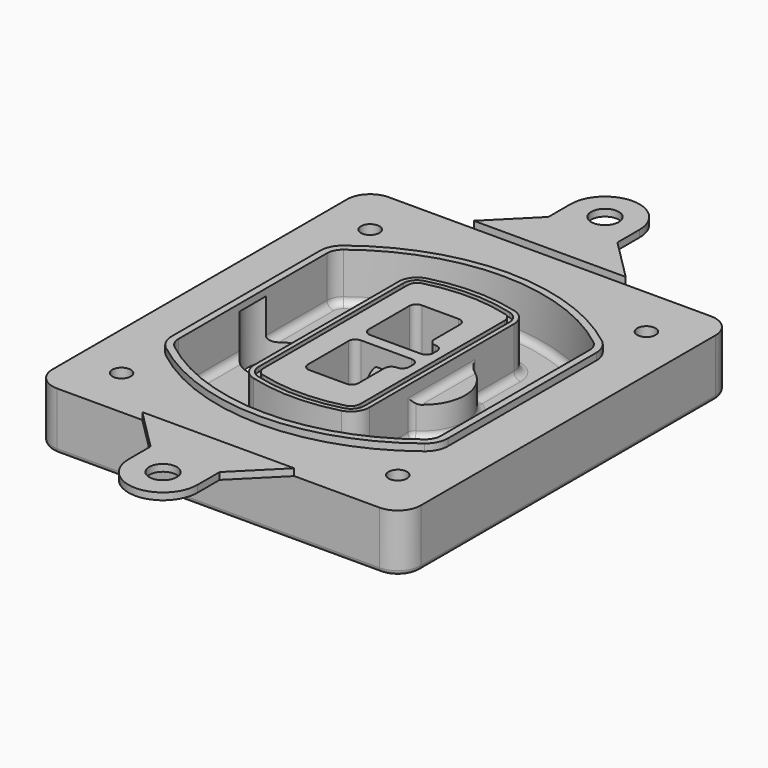
from build123d import *

# Parameters (mm, degrees)
F0_R      = 4
F1_DEPTH  = 25
F2_DEPTH  = 3
F3_DEPTH  = 18
F5_DEPTH  = 21
F6_DEPTH  = 2
F8_DEPTH  = 20
F9_DEPTH  = 16
F10_DEPTH = 25
F7_R      = 6
F7_R_2    = 4
F11_DEPTH = 6
F13_DEPTH = 9
F14_R     = 3
F15_R     = 2
F16_R     = 6
F17_DEPTH = 3
F18_DEPTH = 3


# Not quite as in the source:
# - a feature names something its author has since deleted; it is built from what else it names


with BuildPart() as f1:
    # F0 (on Top) → F1 (new body)
    with BuildSketch(Plane.XY):
        with BuildLine():
            ThreePointArc((-80, -80), (-77.0710678119, -87.0710678119), (-70, -90))
            Line((-70, -90), (70, -90))
            ThreePointArc((70, -90), (77.0710678119, -87.0710678119), (80, -80))
            Line((80, -80), (80, 80))
            ThreePointArc((80, 80), (77.0710678119, 87.0710678119), (70, 90))
            Line((70, 90), (-70, 90))
            ThreePointArc((-70, 90), (-77.0710678119, 87.0710678119), (-80, 80))
            Line((-80, 80), (-80, -80))
        make_face()
        with Locations((-60, -67.5)):
            Circle(F0_R, mode=Mode.SUBTRACT)
        with Locations((60, -67.5)):
            Circle(F0_R, mode=Mode.SUBTRACT)
        with Locations((-60, 67.5)):
            Circle(F0_R, mode=Mode.SUBTRACT)
        with BuildLine():
            ThreePointArc((-64, 40.2934422872), (-62.5820384798, 46.4328484224), (-58.6153846154, 51.3286200352))
            ThreePointArc((-58.6153846154, 51.3286200352), (0, 71.5), (58.6153846154, 51.3286200352))
            ThreePointArc((58.6153846154, 51.3286200352), (62.5820384798, 46.4328484224), (64, 40.2934422872))
            Line((64, 40.2934422872), (64, -40.2934422872))
            ThreePointArc((64, -40.2934422872), (62.5820384798, -46.4328484224), (58.6153846154, -51.3286200352))
            ThreePointArc((58.6153846154, -51.3286200352), (0, -71.5), (-58.6153846154, -51.3286200352))
            ThreePointArc((-58.6153846154, -51.3286200352), (-62.5820384798, -46.4328484224), (-64, -40.2934422872))
            Line((-64, -40.2934422872), (-64, 40.2934422872))
        make_face(mode=Mode.SUBTRACT)
        with Locations((60, 67.5)):
            Circle(F0_R, mode=Mode.SUBTRACT)
        with BuildLine():
            ThreePointArc((58.6153846154, 51.3286200352), (0, 71.5), (-58.6153846154, 51.3286200352))
            ThreePointArc((-58.6153846154, 51.3286200352), (-62.5820384798, 46.4328484224), (-64, 40.2934422872))
            Line((-64, 40.2934422872), (-64, -40.2934422872))
            ThreePointArc((-64, -40.2934422872), (-62.5820384798, -46.4328484224), (-58.6153846154, -51.3286200352))
            ThreePointArc((-58.6153846154, -51.3286200352), (0, -71.5), (58.6153846154, -51.3286200352))
            ThreePointArc((58.6153846154, -51.3286200352), (62.5820384798, -46.4328484224), (64, -40.2934422872))
            Line((64, -40.2934422872), (64, 40.2934422872))
            ThreePointArc((64, 40.2934422872), (62.5820384798, 46.4328484224), (58.6153846154, 51.3286200352))
        make_face()
        with BuildLine():
            Line((-60, -40.2934422872), (-60, 40.2934422872))
            ThreePointArc((-60, 40.2934422872), (-58.9871703427, 44.6787323838), (-56.1538461538, 48.1757121072))
            ThreePointArc((-56.1538461538, 48.1757121072), (0, 67.5), (56.1538461538, 48.1757121072))
            ThreePointArc((56.1538461538, 48.1757121072), (58.9871703427, 44.6787323838), (60, 40.2934422872))
            Line((60, 40.2934422872), (60, -40.2934422872))
            ThreePointArc((60, -40.2934422872), (58.9871703427, -44.6787323838), (56.1538461538, -48.1757121072))
            ThreePointArc((56.1538461538, -48.1757121072), (0, -67.5), (-56.1538461538, -48.1757121072))
            ThreePointArc((-56.1538461538, -48.1757121072), (-58.9871703427, -44.6787323838), (-60, -40.2934422872))
        make_face(mode=Mode.SUBTRACT)
        with BuildLine():
            ThreePointArc((-56.1538461538, 48.1757121072), (-58.9871703427, 44.6787323838), (-60, 40.2934422872))
            Line((-60, 40.2934422872), (-60, -40.2934422872))
            ThreePointArc((-60, -40.2934422872), (-58.9871703427, -44.6787323838), (-56.1538461538, -48.1757121072))
            ThreePointArc((-56.1538461538, -48.1757121072), (0, -67.5), (56.1538461538, -48.1757121072))
            ThreePointArc((56.1538461538, -48.1757121072), (58.9871703427, -44.6787323838), (60, -40.2934422872))
            Line((60, -40.2934422872), (60, 40.2934422872))
            ThreePointArc((60, 40.2934422872), (58.9871703427, 44.6787323838), (56.1538461538, 48.1757121072))
            ThreePointArc((56.1538461538, 48.1757121072), (0, 67.5), (-56.1538461538, 48.1757121072))
        make_face()
        with BuildLine():
            ThreePointArc((54.3076923077, 45.8110311612), (56.2910192399, 43.3631453548), (57, 40.2934422872))
            Line((57, 40.2934422872), (57, -40.2934422872))
            ThreePointArc((57, -40.2934422872), (56.2910192399, -43.3631453548), (54.3076923077, -45.8110311612))
            ThreePointArc((54.3076923077, -45.8110311612), (0, -64.5), (-54.3076923077, -45.8110311612))
            ThreePointArc((-54.3076923077, -45.8110311612), (-56.2910192399, -43.3631453548), (-57, -40.2934422872))
            Line((-57, -40.2934422872), (-57, 40.2934422872))
            ThreePointArc((-57, 40.2934422872), (-56.2910192399, 43.3631453548), (-54.3076923077, 45.8110311612))
            ThreePointArc((-54.3076923077, 45.8110311612), (0, 64.5), (54.3076923077, 45.8110311612))
        make_face(mode=Mode.SUBTRACT)
        with BuildLine():
            Line((57, -40.2934422872), (57, 40.2934422872))
            ThreePointArc((57, 40.2934422872), (56.2910192399, 43.3631453548), (54.3076923077, 45.8110311612))
            ThreePointArc((54.3076923077, 45.8110311612), (0, 64.5), (-54.3076923077, 45.8110311612))
            ThreePointArc((-54.3076923077, 45.8110311612), (-56.2910192399, 43.3631453548), (-57, 40.2934422872))
            Line((-57, 40.2934422872), (-57, -40.2934422872))
            ThreePointArc((-57, -40.2934422872), (-56.2910192399, -43.3631453548), (-54.3076923077, -45.8110311612))
            ThreePointArc((-54.3076923077, -45.8110311612), (0, -64.5), (54.3076923077, -45.8110311612))
            ThreePointArc((54.3076923077, -45.8110311612), (56.2910192399, -43.3631453548), (57, -40.2934422872))
        make_face()
    extrude(amount=-F1_DEPTH)

    # F0 (on Top) → F2 (join)
    with BuildSketch(Plane.XY):
        with BuildLine():
            ThreePointArc((-56.1538461538, 48.1757121072), (-58.9871703427, 44.6787323838), (-60, 40.2934422872))
            Line((-60, 40.2934422872), (-60, -40.2934422872))
            ThreePointArc((-60, -40.2934422872), (-58.9871703427, -44.6787323838), (-56.1538461538, -48.1757121072))
            ThreePointArc((-56.1538461538, -48.1757121072), (0, -67.5), (56.1538461538, -48.1757121072))
            ThreePointArc((56.1538461538, -48.1757121072), (58.9871703427, -44.6787323838), (60, -40.2934422872))
            Line((60, -40.2934422872), (60, 40.2934422872))
            ThreePointArc((60, 40.2934422872), (58.9871703427, 44.6787323838), (56.1538461538, 48.1757121072))
            ThreePointArc((56.1538461538, 48.1757121072), (0, 67.5), (-56.1538461538, 48.1757121072))
        make_face()
        with BuildLine():
            ThreePointArc((54.3076923077, 45.8110311612), (56.2910192399, 43.3631453548), (57, 40.2934422872))
            Line((57, 40.2934422872), (57, -40.2934422872))
            ThreePointArc((57, -40.2934422872), (56.2910192399, -43.3631453548), (54.3076923077, -45.8110311612))
            ThreePointArc((54.3076923077, -45.8110311612), (0, -64.5), (-54.3076923077, -45.8110311612))
            ThreePointArc((-54.3076923077, -45.8110311612), (-56.2910192399, -43.3631453548), (-57, -40.2934422872))
            Line((-57, -40.2934422872), (-57, 40.2934422872))
            ThreePointArc((-57, 40.2934422872), (-56.2910192399, 43.3631453548), (-54.3076923077, 45.8110311612))
            ThreePointArc((-54.3076923077, 45.8110311612), (0, 64.5), (54.3076923077, 45.8110311612))
        make_face(mode=Mode.SUBTRACT)
    extrude(amount=F2_DEPTH)

    # F0 (on Top) → F3 (cut)
    with BuildSketch(Plane.XY):
        with BuildLine():
            Line((57, -40.2934422872), (57, 40.2934422872))
            ThreePointArc((57, 40.2934422872), (56.2910192399, 43.3631453548), (54.3076923077, 45.8110311612))
            ThreePointArc((54.3076923077, 45.8110311612), (0, 64.5), (-54.3076923077, 45.8110311612))
            ThreePointArc((-54.3076923077, 45.8110311612), (-56.2910192399, 43.3631453548), (-57, 40.2934422872))
            Line((-57, 40.2934422872), (-57, -40.2934422872))
            ThreePointArc((-57, -40.2934422872), (-56.2910192399, -43.3631453548), (-54.3076923077, -45.8110311612))
            ThreePointArc((-54.3076923077, -45.8110311612), (0, -64.5), (54.3076923077, -45.8110311612))
            ThreePointArc((54.3076923077, -45.8110311612), (56.2910192399, -43.3631453548), (57, -40.2934422872))
        make_face()
    extrude(amount=-F3_DEPTH, mode=Mode.SUBTRACT)

    # F4 (on face) → F5 (join, through all)
    with BuildSketch(Plane.XY.offset(3)):
        with BuildLine():
            ThreePointArc((-25, -39.2465276821), (-23.3511545998, -44.1109737193), (-19.0842911877, -46.9702398883))
            ThreePointArc((-19.0842911877, -46.9702398883), (0, -49.5), (19.0842911877, -46.9702398883))
            ThreePointArc((19.0842911877, -46.9702398883), (23.3511545998, -44.1109737193), (25, -39.2465276821))
            Line((25, -39.2465276821), (25, 39.2465276821))
            ThreePointArc((25, 39.2465276821), (23.3511545998, 44.1109737193), (19.0842911877, 46.9702398883))
            ThreePointArc((19.0842911877, 46.9702398883), (0, 49.5), (-19.0842911877, 46.9702398883))
            ThreePointArc((-19.0842911877, 46.9702398883), (-23.3511545998, 44.1109737193), (-25, 39.2465276821))
            Line((-25, 39.2465276821), (-25, -39.2465276821))
        make_face()
        with BuildLine():
            ThreePointArc((18.5632183908, 45.0393118368), (21.7633659499, 42.89486221), (23, 39.2465276821))
            Line((23, 39.2465276821), (23, -39.2465276821))
            ThreePointArc((23, -39.2465276821), (21.7633659499, -42.89486221), (18.5632183908, -45.0393118368))
            ThreePointArc((18.5632183908, -45.0393118368), (0, -47.5), (-18.5632183908, -45.0393118368))
            ThreePointArc((-18.5632183908, -45.0393118368), (-21.7633659499, -42.89486221), (-23, -39.2465276821))
            Line((-23, -39.2465276821), (-23, 39.2465276821))
            ThreePointArc((-23, 39.2465276821), (-21.7633659499, 42.89486221), (-18.5632183908, 45.0393118368))
            ThreePointArc((-18.5632183908, 45.0393118368), (0, 47.5), (18.5632183908, 45.0393118368))
        make_face(mode=Mode.SUBTRACT)
        with BuildLine():
            Line((23, -39.2465276821), (23, 39.2465276821))
            ThreePointArc((23, 39.2465276821), (21.7633659499, 42.89486221), (18.5632183908, 45.0393118368))
            ThreePointArc((18.5632183908, 45.0393118368), (0, 47.5), (-18.5632183908, 45.0393118368))
            ThreePointArc((-18.5632183908, 45.0393118368), (-21.7633659499, 42.89486221), (-23, 39.2465276821))
            Line((-23, 39.2465276821), (-23, -39.2465276821))
            ThreePointArc((-23, -39.2465276821), (-21.7633659499, -42.89486221), (-18.5632183908, -45.0393118368))
            ThreePointArc((-18.5632183908, -45.0393118368), (0, -47.5), (18.5632183908, -45.0393118368))
            ThreePointArc((18.5632183908, -45.0393118368), (21.7633659499, -42.89486221), (23, -39.2465276821))
        make_face()
        with BuildLine():
            ThreePointArc((18.0421455939, 43.1083837852), (20.1755772999, 41.6787507007), (21, 39.2465276821))
            Line((21, 39.2465276821), (21, -39.2465276821))
            ThreePointArc((21, -39.2465276821), (20.1755772999, -41.6787507007), (18.0421455939, -43.1083837852))
            ThreePointArc((18.0421455939, -43.1083837852), (0, -45.5), (-18.0421455939, -43.1083837852))
            ThreePointArc((-18.0421455939, -43.1083837852), (-20.1755772999, -41.6787507007), (-21, -39.2465276821))
            Line((-21, -39.2465276821), (-21, 39.2465276821))
            ThreePointArc((-21, 39.2465276821), (-20.1755772999, 41.6787507007), (-18.0421455939, 43.1083837852))
            ThreePointArc((-18.0421455939, 43.1083837852), (0, 45.5), (18.0421455939, 43.1083837852))
        make_face(mode=Mode.SUBTRACT)
        with BuildLine():
            Line((21, -39.2465276821), (21, 39.2465276821))
            ThreePointArc((21, 39.2465276821), (20.1755772999, 41.6787507007), (18.0421455939, 43.1083837852))
            ThreePointArc((18.0421455939, 43.1083837852), (0, 45.5), (-18.0421455939, 43.1083837852))
            ThreePointArc((-18.0421455939, 43.1083837852), (-20.1755772999, 41.6787507007), (-21, 39.2465276821))
            Line((-21, 39.2465276821), (-21, -39.2465276821))
            ThreePointArc((-21, -39.2465276821), (-20.1755772999, -41.6787507007), (-18.0421455939, -43.1083837852))
            ThreePointArc((-18.0421455939, -43.1083837852), (0, -45.5), (18.0421455939, -43.1083837852))
            ThreePointArc((18.0421455939, -43.1083837852), (20.1755772999, -41.6787507007), (21, -39.2465276821))
        make_face()
        with BuildLine():
            Line((-8, -2.5), (14, -2.5))
            ThreePointArc((14, -2.5), (16.1213203436, -3.3786796564), (17, -5.5))
            Line((17, -5.5), (17, -7.5))
            ThreePointArc((17, -7.5), (16.1213203436, -9.6213203436), (14, -10.5))
            ThreePointArc((14, -10.5), (11.8786796564, -11.3786796564), (11, -13.5))
            Line((11, -13.5), (11, -27.5))
            ThreePointArc((11, -27.5), (10.1213203436, -29.6213203436), (8, -30.5))
            Line((8, -30.5), (-8, -30.5))
            ThreePointArc((-8, -30.5), (-10.1213203436, -29.6213203436), (-11, -27.5))
            Line((-11, -27.5), (-11, -5.5))
            ThreePointArc((-11, -5.5), (-10.1213203436, -3.3786796564), (-8, -2.5))
        make_face(mode=Mode.SUBTRACT)
        with BuildLine():
            ThreePointArc((-8, 2.5), (-10.1213203436, 3.3786796564), (-11, 5.5))
            Line((-11, 5.5), (-11, 27.5))
            ThreePointArc((-11, 27.5), (-10.1213203436, 29.6213203436), (-8, 30.5))
            Line((-8, 30.5), (8, 30.5))
            ThreePointArc((8, 30.5), (10.1213203436, 29.6213203436), (11, 27.5))
            Line((11, 27.5), (11, 13.5))
            ThreePointArc((11, 13.5), (11.8786796564, 11.3786796564), (14, 10.5))
            ThreePointArc((14, 10.5), (16.1213203436, 9.6213203436), (17, 7.5))
            Line((17, 7.5), (17, 5.5))
            ThreePointArc((17, 5.5), (16.1213203436, 3.3786796564), (14, 2.5))
            Line((14, 2.5), (-8, 2.5))
        make_face(mode=Mode.SUBTRACT)
    extrude(amount=-F5_DEPTH)

    # F4 (on face) → F6 (cut)
    with BuildSketch(Plane.XY.offset(3)):
        with BuildLine():
            Line((23, -39.2465276821), (23, 39.2465276821))
            ThreePointArc((23, 39.2465276821), (21.7633659499, 42.89486221), (18.5632183908, 45.0393118368))
            ThreePointArc((18.5632183908, 45.0393118368), (0, 47.5), (-18.5632183908, 45.0393118368))
            ThreePointArc((-18.5632183908, 45.0393118368), (-21.7633659499, 42.89486221), (-23, 39.2465276821))
            Line((-23, 39.2465276821), (-23, -39.2465276821))
            ThreePointArc((-23, -39.2465276821), (-21.7633659499, -42.89486221), (-18.5632183908, -45.0393118368))
            ThreePointArc((-18.5632183908, -45.0393118368), (0, -47.5), (18.5632183908, -45.0393118368))
            ThreePointArc((18.5632183908, -45.0393118368), (21.7633659499, -42.89486221), (23, -39.2465276821))
        make_face()
        with BuildLine():
            ThreePointArc((18.0421455939, 43.1083837852), (20.1755772999, 41.6787507007), (21, 39.2465276821))
            Line((21, 39.2465276821), (21, -39.2465276821))
            ThreePointArc((21, -39.2465276821), (20.1755772999, -41.6787507007), (18.0421455939, -43.1083837852))
            ThreePointArc((18.0421455939, -43.1083837852), (0, -45.5), (-18.0421455939, -43.1083837852))
            ThreePointArc((-18.0421455939, -43.1083837852), (-20.1755772999, -41.6787507007), (-21, -39.2465276821))
            Line((-21, -39.2465276821), (-21, 39.2465276821))
            ThreePointArc((-21, 39.2465276821), (-20.1755772999, 41.6787507007), (-18.0421455939, 43.1083837852))
            ThreePointArc((-18.0421455939, 43.1083837852), (0, 45.5), (18.0421455939, 43.1083837852))
        make_face(mode=Mode.SUBTRACT)
    extrude(amount=-F6_DEPTH, mode=Mode.SUBTRACT)

    # F7 (on face) → F8 (join)
    with BuildSketch(Plane(origin=(0, 0, -25), x_dir=(1, 0, 0), z_dir=(0, 0, -1))):
        with BuildLine():
            ThreePointArc((3.28842436, 0), (16.7567035675, 13.4682792075), (30.224982775, 0))
            Line((30.224982775, 0), (35.224982775, 0))
            ThreePointArc((35.224982775, 0), (16.7567035675, 18.4682792075), (-1.71157564, 0))
            Line((-1.71157564, 0), (3.28842436, 0))
        make_face()
        with BuildLine():
            Line((3.28842436, 0), (30.224982775, 0))
            ThreePointArc((30.224982775, 0), (16.7567035675, 13.4682792075), (3.28842436, 0))
        make_face()
        with BuildLine():
            ThreePointArc((3.28842436, 0), (16.7567035675, -13.4682792075), (30.224982775, 0))
            Line((30.224982775, 0), (3.28842436, 0))
        make_face()
        with BuildLine():
            Line((35.224982775, 0), (30.224982775, 0))
            ThreePointArc((30.224982775, 0), (16.7567035675, -13.4682792075), (3.28842436, 0))
            Line((3.28842436, 0), (-1.71157564, 0))
            ThreePointArc((-1.71157564, 0), (16.7567035675, -18.4682792075), (35.224982775, 0))
        make_face()
    extrude(amount=-F8_DEPTH)

    # F7 (on face) → F9 (cut)
    with BuildSketch(Plane(origin=(0, 0, -25), x_dir=(1, 0, 0), z_dir=(0, 0, -1))):
        with BuildLine():
            Line((3.28842436, 0), (30.224982775, 0))
            ThreePointArc((30.224982775, 0), (16.7567035675, 13.4682792075), (3.28842436, 0))
        make_face()
        with BuildLine():
            ThreePointArc((3.28842436, 0), (16.7567035675, -13.4682792075), (30.224982775, 0))
            Line((30.224982775, 0), (3.28842436, 0))
        make_face()
    extrude(amount=-F9_DEPTH, mode=Mode.SUBTRACT)

    # F7 (on face) → F10 (cut)
    with BuildSketch(Plane(origin=(0, 0, -25), x_dir=(1, 0, 0), z_dir=(0, 0, -1))):
        with BuildLine():
            Line((-59.0318229325, 0), (-32.0952645175, 0))
            ThreePointArc((-32.0952645175, 0), (-45.563543725, 13.4682792075), (-59.0318229325, 0))
        make_face()
        with BuildLine():
            ThreePointArc((-59.0318229325, 0), (-45.563543725, -13.4682792075), (-32.0952645175, 0))
            Line((-32.0952645175, 0), (-59.0318229325, 0))
        make_face()
    extrude(amount=-F10_DEPTH, mode=Mode.SUBTRACT)

    # F7 (on face) → F11 (cut)
    with BuildSketch(Plane(origin=(0, 0, -25), x_dir=(1, 0, 0), z_dir=(0, 0, -1))):
        with Locations((60, -67.5)):
            Circle(F7_R)
        with Locations((60, -67.5)):
            Circle(F7_R_2, mode=Mode.SUBTRACT)
        with Locations((-60, -67.5)):
            Circle(F7_R)
        with Locations((-60, -67.5)):
            Circle(F7_R_2, mode=Mode.SUBTRACT)
        with Locations((-60, 67.5)):
            Circle(F7_R)
        with Locations((-60, 67.5)):
            Circle(F7_R_2, mode=Mode.SUBTRACT)
        with Locations((60, 67.5)):
            Circle(F7_R)
        with Locations((60, 67.5)):
            Circle(F7_R_2, mode=Mode.SUBTRACT)
    extrude(amount=-F11_DEPTH, mode=Mode.SUBTRACT)

    # F12 (on face) → F13 (cut, through all)
    with BuildSketch(Plane(origin=(0, 0, -9), x_dir=(1, 0, 0), z_dir=(0, 0, -1))):
        with BuildLine():
            Line((11, 13.5), (11, 17.5481537753))
            ThreePointArc((11, 17.5481537753), (2.5696536419, 11.8239143813), (-1.5415842455, 2.5))
            Line((-1.5415842455, 2.5), (3.5224848595, 2.5))
            ThreePointArc((3.5224848595, 2.5), (6.1857188154, 8.3455872281), (11.2536447004, 12.2927168648))
            ThreePointArc((11.2536447004, 12.2927168648), (11.0640958889, 12.8831798879), (11, 13.5))
        make_face()
        with BuildLine():
            ThreePointArc((11.2536447004, -12.2927168648), (6.1857188154, -8.3455872281), (3.5224848595, -2.5))
            Line((3.5224848595, -2.5), (-1.5415842455, -2.5))
            ThreePointArc((-1.5415842455, -2.5), (2.5696536419, -11.8239143813), (11, -17.5481537753))
            Line((11, -17.5481537753), (11, -13.5))
            ThreePointArc((11, -13.5), (11.0640958889, -12.8831798879), (11.2536447004, -12.2927168648))
        make_face()
        with BuildLine():
            ThreePointArc((11.2536447004, 12.2927168648), (6.1857188154, 8.3455872281), (3.5224848595, 2.5))
            Line((3.5224848595, 2.5), (14, 2.5))
            ThreePointArc((14, 2.5), (16.1213203436, 3.3786796564), (17, 5.5))
            Line((17, 5.5), (17, 7.5))
            ThreePointArc((17, 7.5), (16.1213203436, 9.6213203436), (14, 10.5))
            ThreePointArc((14, 10.5), (12.3601599782, 10.9878446101), (11.2536447004, 12.2927168648))
        make_face()
        with BuildLine():
            Line((14, -2.5), (3.5224848595, -2.5))
            ThreePointArc((3.5224848595, -2.5), (6.1857188154, -8.3455872281), (11.2536447004, -12.2927168648))
            ThreePointArc((11.2536447004, -12.2927168648), (12.3601599782, -10.9878446101), (14, -10.5))
            ThreePointArc((14, -10.5), (16.1213203436, -9.6213203436), (17, -7.5))
            Line((17, -7.5), (17, -5.5))
            ThreePointArc((17, -5.5), (16.1213203436, -3.3786796564), (14, -2.5))
        make_face()
    extrude(amount=F13_DEPTH, mode=Mode.SUBTRACT)

    # F14
    f14_edges = [f1.edges().sort_by_distance(p)[0] for p in [
        (-57, -23.703476, -18),
        (-57, 23.703476, -18),
        (25, 0, -5),
        (25, 16.526506, -11.5),
        (25, -16.526506, -11.5),
        (25, -27.886517, -18),
        (35.224983, 0, -18),
    ]]
    fillet(f14_edges, radius=F14_R)

    # F15
    f15_edges = [f1.edges().sort_by_distance(p)[0] for p in [
        (0, -90, -25),
    ]]
    fillet(f15_edges, radius=F15_R)


with BuildPart() as f17:
    # F16 (on face) → F17 (new body, through all)
    with BuildSketch(Plane.XY):
        with BuildLine():
            Line((15, 108), (15, 120))
            ThreePointArc((15, 120), (0, 135), (-15, 120))
            Line((-15, 120), (-15, 108))
            Line((-15, 108), (-33, 90))
            Line((-33, 90), (33, 90))
            Line((33, 90), (15, 108))
        make_face()
        with Locations((0, 120)):
            Circle(F16_R, mode=Mode.SUBTRACT)
    extrude(amount=F17_DEPTH)


with BuildPart() as f18:
    # F16 (on face) → F18 (new body, through all)
    with BuildSketch(Plane.XY):
        with BuildLine():
            Line((15, -108), (33, -90))
            Line((33, -90), (-33, -90))
            Line((-33, -90), (-15, -108))
            Line((-15, -108), (-15, -120))
            ThreePointArc((-15, -120), (0, -135), (15, -120))
            Line((15, -120), (15, -108))
        make_face()
        with Locations((0, -120)):
            Circle(F16_R, mode=Mode.SUBTRACT)
    extrude(amount=F18_DEPTH)


solid = Compound([f1.part, f17.part, f18.part])
